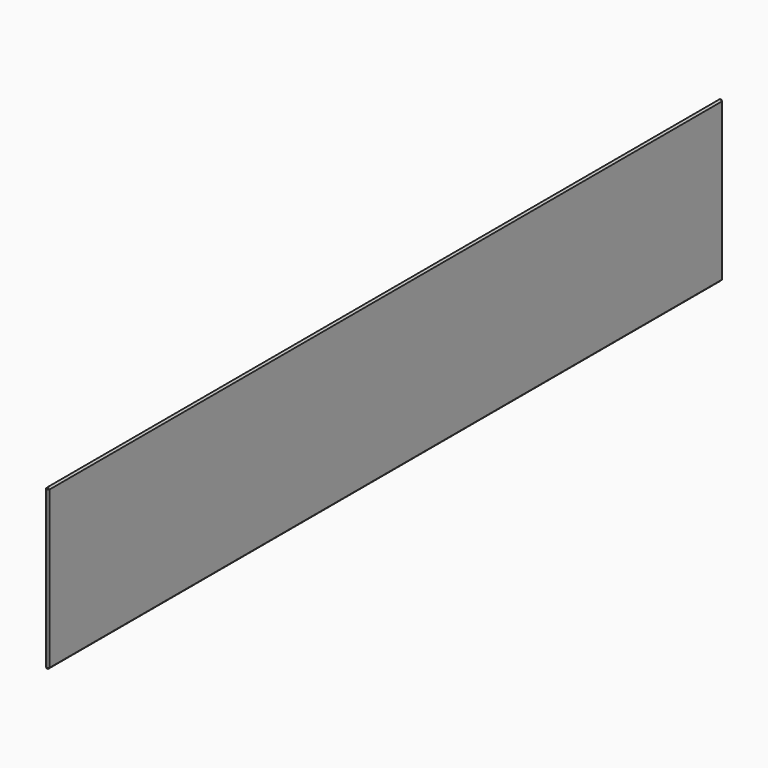
from build123d import *

# Parameters (mm, degrees)
F0_W     = 500
F0_H     = 95
F1_DEPTH = 2
F2_SIZE  = 0.99999


# Not quite as in the source:
# - a fillet or chamfer is up to 0.001 mm smaller than in the source, because OpenCascade refuses the exact size


with BuildPart() as f1:
    # F0 (on Right) → F1 (new body)
    with BuildSketch(Plane.YZ):
        Rectangle(F0_W, F0_H)
    extrude(amount=F1_DEPTH)

    # F2 (size 1 in the source; OpenCascade refuses exactly that, so slightly less here)
    f2_edges = [f1.edges().sort_by_distance(p)[0] for p in [
        (2, 0, 47.5),
        (2, -250, 0),
        (0, -250, 0),
        (0, 0, 47.5),
        (2, 250, 0),
        (0, 0, -47.5),
        (2, 0, -47.5),
        (0, 250, 0),
        (1, 250, 47.5),
        (1, -250, 47.5),
        (1, -250, -47.5),
        (1, 250, -47.5),
    ]]
    chamfer(f2_edges, length=F2_SIZE)


solid = f1.part
